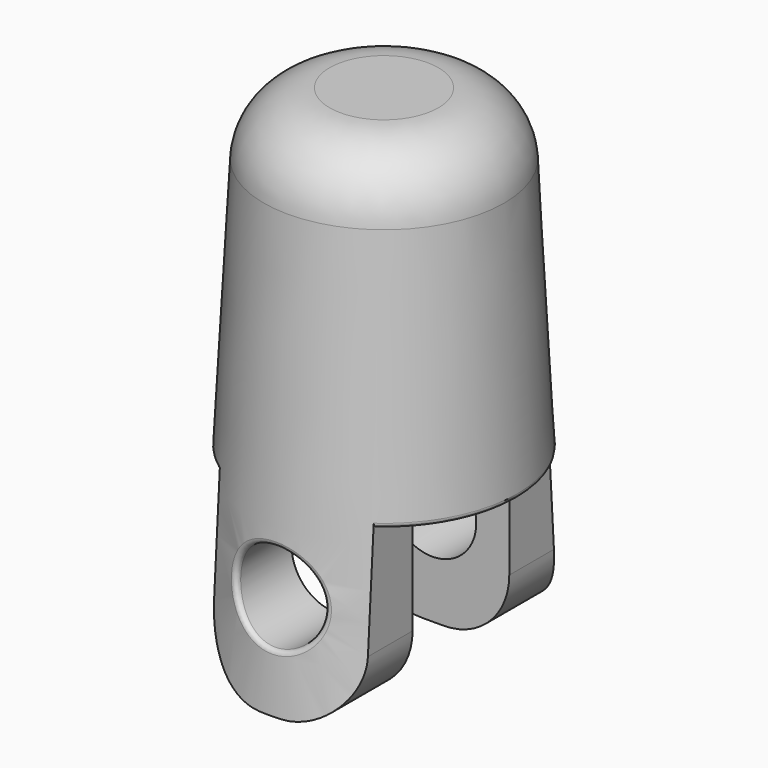
from build123d import *

# Parameters (mm, degrees)
F0_R          = 6.5
F1_DEPTH      = 22.5
F1_TAPER      = 3
F2_R          = 3
F3_W          = 1.5
F3_H          = 5.5
F3_W_2        = 7
F4_DEPTH      = 8
F5_R          = 2
F6_DEPTH      = 25
F6_DEPTH_BACK = 25
F7_T          = 1
F8_R          = 0.2
F9_R          = 3


# Not quite as in the source:
# - a shell that OpenCascade refuses in one call is made with other operations: the cavity is built on its own and cut out


with BuildPart() as f1:
    # F0 (on Top) → F1 (new body)
    with BuildSketch(Plane.XY):
        Circle(F0_R)
    extrude(amount=F1_DEPTH, taper=F1_TAPER)

    # F2
    f2_edges = [f1.edges().sort_by_distance(p)[0] for p in [
        (-5.320825, 0, 22.5),
    ]]
    fillet(f2_edges, radius=F2_R)

    # F3 (on Top) → F4 (cut)
    with BuildSketch(Plane.XY):
        Polygon((5, 2.75), (5, -2.75), (3.5, -2.75), (3.5, -6.25), (6.5, -6.25), (6.5, 6.25), (3.5, 6.25), (3.5, 2.75), align=None)
        with Locations((4.25, 0)):
            Rectangle(F3_W, F3_H)
        Rectangle(F3_W_2, F3_H)
        Polygon((-3.5, -6.25), (-3.5, -2.75), (-5, -2.75), (-5, 2.75), (-3.5, 2.75), (-3.5, 6.25), (-6.5, 6.25), (-6.5, -6.25), align=None)
        with Locations((-4.25, 0)):
            Rectangle(F3_W, F3_H)
    extrude(amount=F4_DEPTH, mode=Mode.SUBTRACT)

    # F5 (on face) → F6 (cut, two sides)
    with BuildSketch(Plane(origin=(0, -2.75, 0), x_dir=(-1, 0, 0), z_dir=(0, 1, 0))) as f6_sk:
        with Locations((0, 4.5984359458)):
            Circle(F5_R)
    extrude(amount=F6_DEPTH, mode=Mode.SUBTRACT)
    extrude(f6_sk.sketch, amount=-F6_DEPTH_BACK, mode=Mode.SUBTRACT)

    # F7: shell of thickness 1, made by hand


with BuildPart() as f7_core1:
    # F7_t2: copy of F1
    add(f1.part)

    # the walls: a layer under each face that stays
    f7_faces = [f7_core1.faces().sort_by_distance(p)[0] for p in [
        (-5.9849099351, 0, 9.8285039344),
        (3.5, -4.1136127875, 4),
        (0, -4.625, 0),
        (-3.5, -4.1136127875, 4),
        (-3.5, 4.1136127875, 4),
        (0, 4.625, 0),
        (3.5, 4.1136127875, 4),
        (-4.5389949931, 0, 21.676123113),
        (2, 4.5569343282, 4.5984359458),
        (2, -4.5569343282, 4.5984359458),
        (-2.3333333333, -2.75, 6.6666666667),
        (2.3333333333, 2.75, 6.6666666667),
        (0, 0, 22.5),
    ]]
    thicken(f7_faces, amount=-F7_T, mode=Mode.SUBTRACT)


with BuildPart() as f1_1:
    add(f1.part)

    # what is left inside the walls is the cavity
    f7_cavity = [f7_core1.part.solids().sort_by_distance(p)[0] for p in [
        (0, -4.859979, 1.588436),
        (-4.927561, 0, 10.705533),
        (0, 4.859979, 1.588436),
    ]]
    add(f7_cavity, mode=Mode.SUBTRACT)

    # F8
    f8_edges = [f1_1.edges().sort_by_distance(p)[0] for p in [
        (1.999873, -5.932154, 4.575894),
        (5.397127, -2.801142, 8),
        (-6.080738, 0, 8),
        (5.397127, 2.801142, 8),
        (1.999882, 5.932105, 4.576739),
    ]]
    fillet(f8_edges, radius=F8_R)

    # F9
    f9_edges = [f1_1.edges().sort_by_distance(p)[0] for p in [
        (3.5, -4.113613, 0),
        (3.5, 4.113613, 0),
        (-3.5, 4.113613, 0),
        (-3.5, -4.113613, 0),
    ]]
    fillet(f9_edges, radius=F9_R)


solid = f1_1.part
